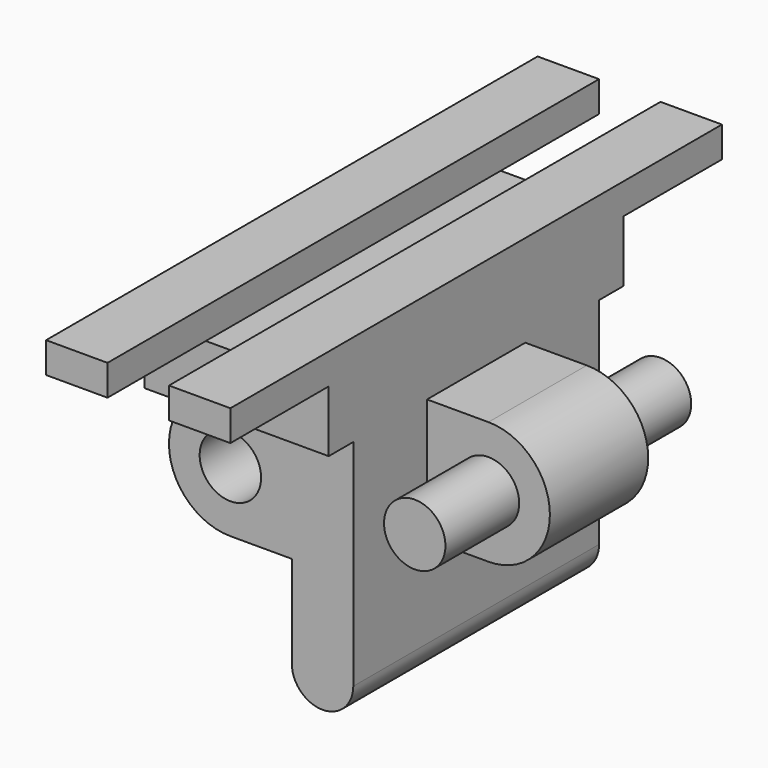
from build123d import *

# Parameters (mm, degrees)
F0_W      = 5
F0_H      = 10
F0_R      = 2.5
F1_DEPTH  = 12.5
F2_DEPTH  = 5
F3_DEPTH  = 12.5
F4_DEPTH  = 7.5
F7_DEPTH  = 10
F8_R      = 2.5
F9_R      = 2.49999
F10_W     = 15
F10_H     = 30
F11_DEPTH = 5
F12_W     = 5
F12_H     = 50
F13_DEPTH = 2.5


# Not quite as in the source:
# - a fillet or chamfer is up to 0.001 mm smaller than in the source, because OpenCascade refuses the exact size


with BuildPart() as f1:
    # F0 (on Front) → F1 (new body)
    with BuildSketch(Plane.XZ):
        with Locations((7.5, 0)):
            Rectangle(F0_W, F0_H)
        with BuildLine():
            Line((5, 5), (0, 5))
            ThreePointArc((0, 5), (-5, 0), (0, -5))
            Line((0, -5), (5, -5))
            Line((5, -5), (5, 5))
        make_face()
        Circle(F0_R, mode=Mode.SUBTRACT)
    extrude(amount=F1_DEPTH)

    # F0 (on Front) → F2 (join)
    with BuildSketch(Plane.XZ):
        with BuildLine():
            Line((15, 5), (10, 5))
            Line((10, 5), (10, -5))
            Line((10, -5), (15, -5))
            ThreePointArc((15, -5), (20, 0), (15, 5))
        make_face()
        with Locations((15, 0)):
            Circle(F0_R, mode=Mode.SUBTRACT)
    extrude(amount=F2_DEPTH)

    # F0 (on Front) → F3 (join)
    with BuildSketch(Plane.XZ):
        with Locations((15, 0)):
            Circle(F0_R)
    extrude(amount=F3_DEPTH)

    # F0 (on Front) → F4 (cut)
    with BuildSketch(Plane.XZ):
        with BuildLine():
            Line((5, 5), (0, 5))
            ThreePointArc((0, 5), (-5, 0), (0, -5))
            Line((0, -5), (5, -5))
            Line((5, -5), (5, 5))
        make_face()
        Circle(F0_R, mode=Mode.SUBTRACT)
    extrude(amount=F4_DEPTH, mode=Mode.SUBTRACT)

    # F5: F1 across plane


with BuildPart() as f1_1:
    add(f1.part)
    add(f1.part.mirror(Plane.XZ))

    # F6 (on face) → F7 (join)
    with BuildSketch(Plane(origin=(0, 0, -5), x_dir=(1, 0, 0), z_dir=(0, 0, -1))):
        Polygon((10, 5), (10, 12.5), (5, 12.5), (5, 7.5), (5, -7.5), (5, -12.5), (10, -12.5), (10, -5), align=None)
    extrude(amount=F7_DEPTH)

    # F8
    f8_edges = [f1_1.edges().sort_by_distance(p)[0] for p in [
        (10, 0, -15),
    ]]
    fillet(f8_edges, radius=F8_R)

    # F9 (radius 2.5 in the source; OpenCascade refuses exactly that, so slightly less here)
    f9_edges = [f1_1.edges().sort_by_distance(p)[0] for p in [
        (5, 0, -15),
    ]]
    fillet(f9_edges, radius=F9_R)

    # F10 (on face) → F11 (join)
    with BuildSketch(Plane.XY.offset(5)):
        with Locations((2.5, 0)):
            Rectangle(F10_W, F10_H)
    extrude(amount=F11_DEPTH)

    # F12 (on face) → F13 (join)
    with BuildSketch(Plane.XY.offset(10)):
        with Locations((-2.5, 0)):
            Rectangle(F12_W, F12_H)
        with Locations((7.5, 0)):
            Rectangle(F12_W, F12_H)
    extrude(amount=F13_DEPTH)


solid = f1_1.part
